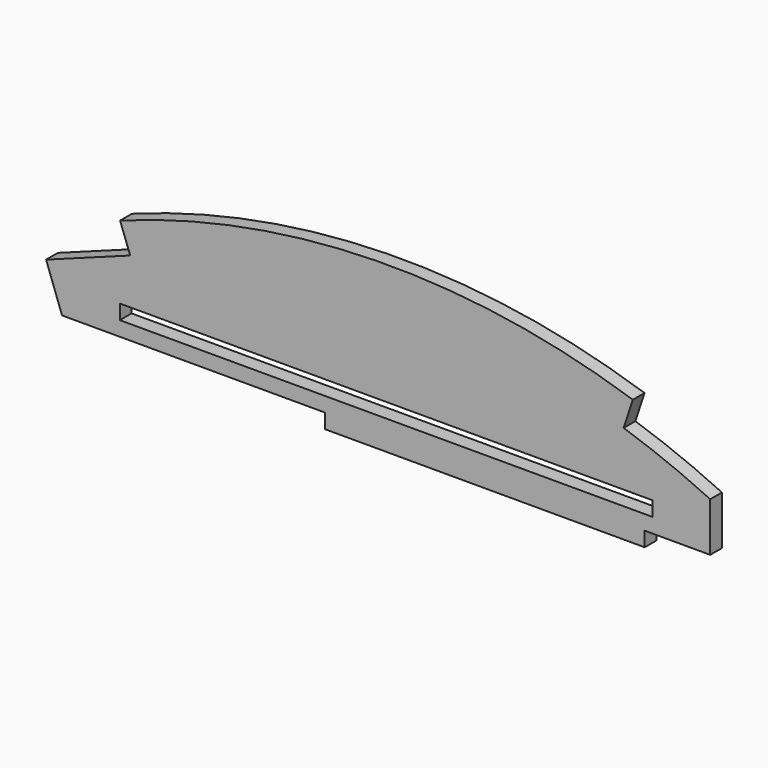
from build123d import *

# Parameters (mm, degrees)
F0_W     = 400
F0_H     = 11
F1_DEPTH = 11


# Not quite as in the source:
# - ends of sketch curves that miss each other by under 0.0002 mm in the source are joined


with BuildPart() as f1:
    # F0 (on Front) → F1 (new body)
    with BuildSketch(Plane.XZ):
        with BuildLine():
            Line((-186.2102279461, 5.2641338535), (-249.389773, -18))
            Line((-249.389773, -18), (-237.378755, -51))
            Line((-237.378755, -51), (-39.805119, -51))
            Line((-39.805119, -51), (-39.805119, -62))
            Line((-39.805119, -62), (200.194881, -62))
            Line((200.194881, -62), (200.194881, -51))
            Line((200.194881, -51), (249.389772, -51))
            Line((249.389772, -51), (249.389772, -14.186388))
            ThreePointArc((249.389772, -14.186388), (217.2940285637, -0.1866284114), (184.3897718043, 11.7900114054))
            Line((184.3897718043, 11.7900114054), (191.267695, 32.687241))
            ThreePointArc((191.267695, 32.687241), (-1.7442805029, 61.9112120177), (-193.620736559, 25.9794888024))
            Line((-193.620736559, 25.9794888024), (-193.812138, 25.909012))
            Line((-193.812138, 25.909012), (-186.2102279461, 5.2641338535))
        make_face()
        with Locations((6.005508, -34.5)):
            Rectangle(F0_W, F0_H, mode=Mode.SUBTRACT)
    extrude(amount=F1_DEPTH)


solid = f1.part
